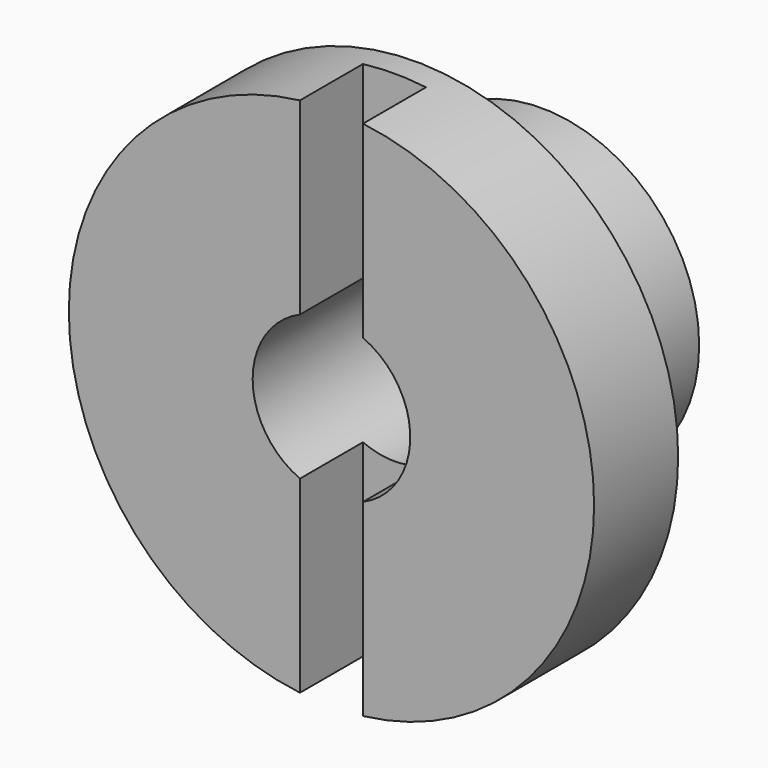
from build123d import *

# Parameters (mm, degrees)
F3_DEPTH = 15
F4_R     = 15
F5_DEPTH = 141
F7_DEPTH = 10


with BuildPart() as f1:
    # F0 (on Top) → F1 (revolve)
    with BuildSketch(Plane.XY):
        Polygon((0, 19.0511253548), (0, -30.9488746452), (50, -30.9488746452), (50, -10.9488746452), (30, -10.9488746452), (30, 19.0511253548), align=None)
    revolve(axis=Axis((0, -5.9488746452, 0), (0, 1, 0)))

    # F2 (on face) → F3 (cut)
    with BuildSketch(Plane.XZ.offset(30.9488746452)):
        with BuildLine():
            ThreePointArc((6, 49.638694584), (0, 50), (-6, 49.638694584))
            Line((-6, 49.638694584), (-6, -49.638694584))
            ThreePointArc((-6, -49.638694584), (0, -50), (6, -49.638694584))
            Line((6, -49.638694584), (6, 49.638694584))
        make_face()
    extrude(amount=-F3_DEPTH, mode=Mode.SUBTRACT)

    # F4 (on face) → F5 (cut)
    with BuildSketch(Plane(origin=(0, 19.0511253548, 0), x_dir=(-1, 0, 0), z_dir=(0, 1, 0))):
        Circle(F4_R)
    extrude(amount=-F5_DEPTH, mode=Mode.SUBTRACT)

    # F6 (on face) → F7 (cut)
    with BuildSketch(Plane(origin=(0, 19.0511253548, 0), x_dir=(-1, 0, 0), z_dir=(0, 1, 0))):
        with BuildLine():
            Line((3, 14.6969384567), (3, 18))
            Line((3, 18), (-3, 18))
            Line((-3, 18), (-3, 14.6969384567))
            ThreePointArc((-3, 14.6969384567), (0, 15), (3, 14.6969384567))
        make_face()
    extrude(amount=-F7_DEPTH, mode=Mode.SUBTRACT)


solid = f1.part
